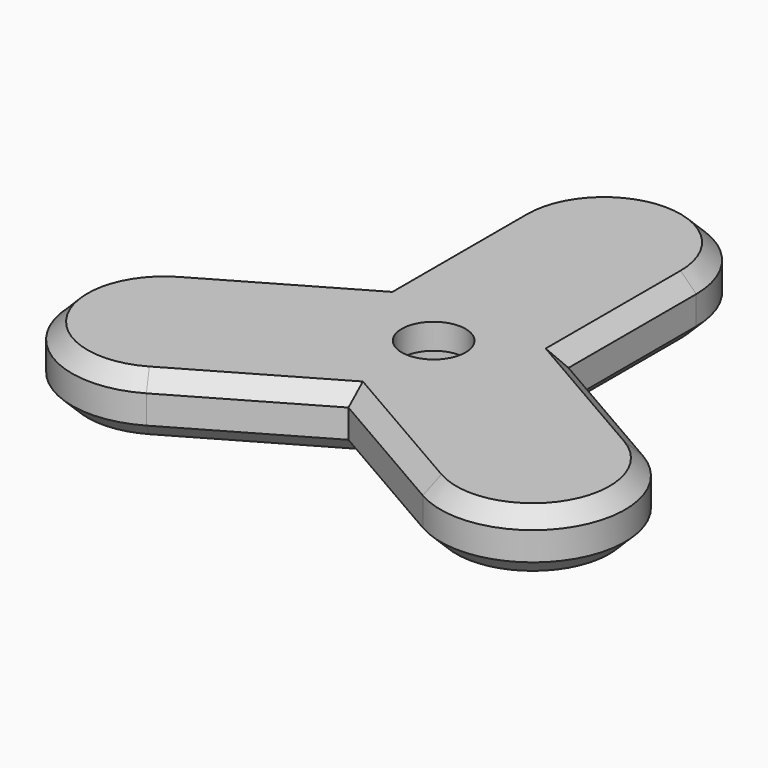
from build123d import *

# Parameters (mm, degrees)
F0_R     = 6.4
F0_R_2   = 4.5
F1_DEPTH = 7.7
F2_DEPTH = 7.9
F3_DEPTH = 4.8
F4_START = 7.7
F4_DEPTH = 0.7
F5_COUNT = 3
F6_SIZE  = 2.2


with BuildPart() as f1:
    # F0 (on Top) → F1 (new body)
    with BuildSketch(Plane.XY):
        with BuildLine():
            ThreePointArc((-13, 0), (0, 13), (13, 0))
            Line((13, 0), (13, 30))
            ThreePointArc((13, 30), (0, 17), (-13, 30))
            Line((-13, 30), (-13, 0))
        make_face()
        with BuildLine():
            ThreePointArc((-13, 30), (0, 17), (13, 30))
            ThreePointArc((13, 30), (0, 43), (-13, 30))
        make_face()
        Polygon((4.9074772881, 38.5), (9.8149545762, 30), (4.9074772881, 21.5), (-4.9074772881, 21.5), (-9.8149545762, 30), (-4.9074772881, 38.5), align=None, mode=Mode.SUBTRACT)
        Polygon((4.9074772881, 21.5), (9.8149545762, 30), (4.9074772881, 38.5), (-4.9074772881, 38.5), (-9.8149545762, 30), (-4.9074772881, 21.5), align=None)
        with BuildLine():
            ThreePointArc((-13, 0), (0, -13), (13, 0))
            ThreePointArc((13, 0), (0, 13), (-13, 0))
        make_face()
        Circle(F0_R, mode=Mode.SUBTRACT)
        Circle(F0_R)
        Circle(F0_R_2, mode=Mode.SUBTRACT)
    extrude(amount=F1_DEPTH)

    # F0 (on Top) → F2 (cut)
    with BuildSketch(Plane.XY):
        Polygon((4.9074772881, 21.5), (9.8149545762, 30), (4.9074772881, 38.5), (-4.9074772881, 38.5), (-9.8149545762, 30), (-4.9074772881, 21.5), align=None)
    extrude(amount=F2_DEPTH, mode=Mode.SUBTRACT)

    # F0 (on Top) → F3 (cut)
    with BuildSketch(Plane.XY):
        Circle(F0_R)
        Circle(F0_R_2, mode=Mode.SUBTRACT)
    extrude(amount=F3_DEPTH, mode=Mode.SUBTRACT)

    # F0 (on Top) → F4 (join)
    with BuildSketch(Plane.XY.offset(F4_START)):
        with BuildLine():
            ThreePointArc((-13, 0), (0, -13), (13, 0))
            ThreePointArc((13, 0), (0, 13), (-13, 0))
        make_face()
        Circle(F0_R, mode=Mode.SUBTRACT)
        with BuildLine():
            ThreePointArc((-13, 30), (0, 17), (13, 30))
            ThreePointArc((13, 30), (0, 43), (-13, 30))
        make_face()
        Polygon((4.9074772881, 38.5), (9.8149545762, 30), (4.9074772881, 21.5), (-4.9074772881, 21.5), (-9.8149545762, 30), (-4.9074772881, 38.5), align=None, mode=Mode.SUBTRACT)
        Polygon((4.9074772881, 21.5), (9.8149545762, 30), (4.9074772881, 38.5), (-4.9074772881, 38.5), (-9.8149545762, 30), (-4.9074772881, 21.5), align=None)
        with BuildLine():
            ThreePointArc((-13, 0), (0, 13), (13, 0))
            Line((13, 0), (13, 30))
            ThreePointArc((13, 30), (0, 17), (-13, 30))
            Line((-13, 30), (-13, 0))
        make_face()
        Circle(F0_R)
        Circle(F0_R_2, mode=Mode.SUBTRACT)
    extrude(amount=F4_DEPTH)

    # F5: F1 ×3 about axis
    f5_axis = Axis((0, 0, 0), (0, 0, -1))


with BuildPart() as f1_1:
    add(f1.part)
    for i in range(1, F5_COUNT):
        add(f1.part.rotate(f5_axis, i * 360 / F5_COUNT))

    # F6
    f6_edges = [f1_1.edges().sort_by_distance(p)[0] for p in [
        (-9.740381, -20.634719, 0),
        (-37.239092, -21.5, 0),
        (-22.740381, 1.881942, 0),
        (22.740381, 1.881942, 0),
        (37.239092, -21.5, 0),
        (9.740381, -20.634719, 0),
        (-13, 18.752777, 0),
        (13, 18.752777, 0),
        (0, 43, 0),
        (13, 18.752777, 8.4),
        (-13, 18.752777, 8.4),
        (-9.740381, -20.634719, 8.4),
        (22.740381, 1.881942, 8.4),
    ]]
    chamfer(f6_edges, length=F6_SIZE)


solid = f1_1.part
